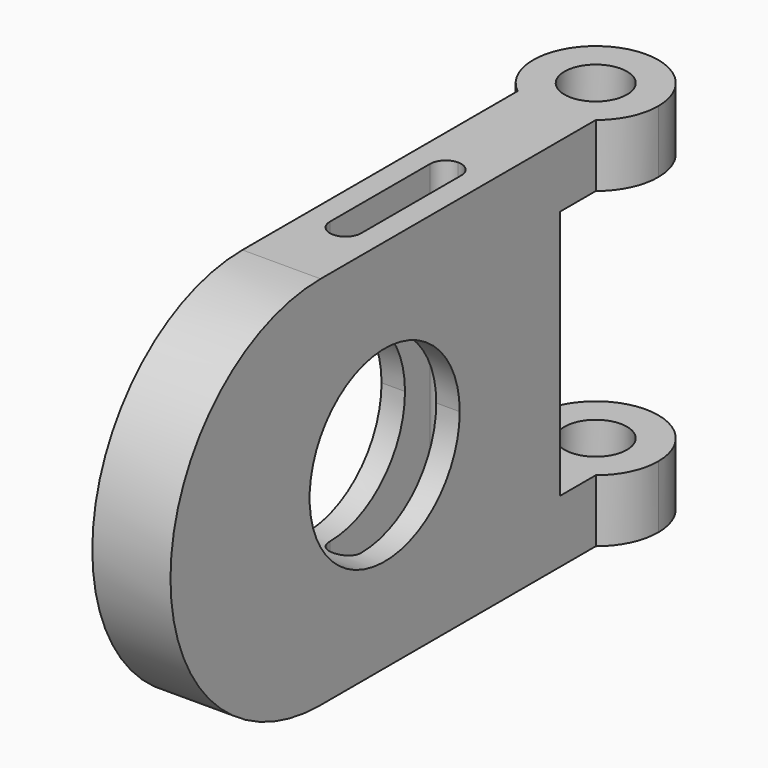
from build123d import *
from build123d import SkipClean  # not in build123d's __all__

# Parameters (mm, degrees)
F1_DEPTH = 152.4
F2_DEPTH = 25.4
F4_DEPTH = 31.75
F5_DEPTH = 41.276
F3_W     = 18.2721313551
F3_H     = 101.6
F6_DEPTH = 41.276
F8_DEPTH = 25.4


with BuildPart() as f1:
    # F0 (on Top) → F1 (new body)
    with BuildSketch(Plane.XY):
        with BuildLine():
            ThreePointArc((15.875, -7.1278686449), (8.4122570223, -11.266516889), (0, -12.7))
            ThreePointArc((0, -12.7), (-8.4122570223, -11.266516889), (-15.875, -7.1278686449))
            Line((-15.875, -7.1278686449), (-15.875, -146.8278686449))
            Line((-15.875, -146.8278686449), (15.875, -146.8278686449))
            Line((15.875, -146.8278686449), (15.875, -7.1278686449))
        make_face()
        with BuildLine():
            ThreePointArc((-6.35, -63.5), (-4.4901280605, -59.0098719395), (0, -57.15))
            ThreePointArc((0, -57.15), (4.4901280605, -59.0098719395), (6.35, -63.5))
            Line((6.35, -63.5), (6.35, -114.3))
            ThreePointArc((6.35, -114.3), (0, -120.65), (-6.35, -114.3))
            Line((-6.35, -114.3), (-6.35, -63.5))
        make_face(mode=Mode.SUBTRACT)
        with BuildLine():
            Line((15.875, -7.1278686449), (0, -7.1278686449))
            Line((0, -7.1278686449), (0, -12.7))
            ThreePointArc((0, -12.7), (8.4122570223, -11.266516889), (15.875, -7.1278686449))
        make_face()
        with BuildLine():
            Line((0, -12.7), (0, -7.1278686449))
            Line((0, -7.1278686449), (-15.875, -7.1278686449))
            ThreePointArc((-15.875, -7.1278686449), (-8.4122570223, -11.266516889), (0, -12.7))
        make_face()
    extrude(amount=-F1_DEPTH)

    # F0 (on Top) → F2 (join)
    with BuildSketch(Plane.XY):
        with BuildLine():
            Line((-15.875, -7.1278686449), (0, -7.1278686449))
            Line((0, -7.1278686449), (15.875, -7.1278686449))
            ThreePointArc((15.875, -7.1278686449), (22.8952505992, 1.7014773719), (25.4, 12.7))
            ThreePointArc((25.4, 12.7), (-10.9985226281, 35.5952505992), (-15.875, -7.1278686449))
        make_face()
        with BuildLine():
            ThreePointArc((12.7, 12.7), (8.9802561211, 3.7197438789), (0, 0))
            ThreePointArc((0, 0), (-8.9802561211, 21.6802561211), (12.7, 12.7))
        make_face(mode=Mode.SUBTRACT)
    extrude(amount=-F2_DEPTH)

    # F3 (on face) → F4 (join)
    with BuildSketch(Plane.YZ.offset(15.875)):
        with BuildLine():
            Line((-146.8278686449, -56.3619617548), (-146.8278686449, 0))
            ThreePointArc((-146.8278686449, 0), (-223.0278686449, -76.2), (-146.8278686449, -152.4))
            Line((-146.8278686449, -152.4), (-146.8278686449, -96.0380382452))
            ThreePointArc((-146.8278686449, -96.0380382452), (-152.4, -76.2), (-146.8278686449, -56.3619617548))
        make_face()
    extrude(amount=-F4_DEPTH)

    # F3 (on face) → F5 (cut, through all)
    with BuildSketch(Plane.YZ.offset(15.875)):
        with BuildLine():
            ThreePointArc((-76.2, -76.2), (-103.9971313551, -39.5194752261), (-146.8278686449, -56.3619617548))
            Line((-146.8278686449, -56.3619617548), (-146.8278686449, -96.0380382452))
            ThreePointArc((-146.8278686449, -96.0380382452), (-103.9971313551, -112.8805247739), (-76.2, -76.2))
        make_face()
    with SkipClean():  # cleaning this boolean's faces spoils the solid; the shape is the same uncleaned
        extrude(amount=-F5_DEPTH, mode=Mode.SUBTRACT)

    # F3 (on face) → F6 (cut, through all)
    with BuildSketch(Plane.YZ.offset(15.875)):
        with Locations((-16.2639343225, -76.2)):
            Rectangle(F3_W, F3_H)
    extrude(amount=-F6_DEPTH, mode=Mode.SUBTRACT)

    # F7 (on face) → F8 (join)
    with BuildSketch(Plane(origin=(0, 0, -152.4), x_dir=(1, 0, 0), z_dir=(0, 0, -1))):
        with BuildLine():
            ThreePointArc((-15.875, 7.1278686449), (-10.9985226281, -35.5952505992), (25.4, -12.7))
            ThreePointArc((25.4, -12.7), (22.8952505992, -1.7014773719), (15.875, 7.1278686449))
            Line((15.875, 7.1278686449), (-15.875, 7.1278686449))
        make_face()
        with BuildLine():
            ThreePointArc((0, 0), (8.9802561211, -3.7197438789), (12.7, -12.7))
            ThreePointArc((12.7, -12.7), (-8.9802561211, -21.6802561211), (0, 0))
        make_face(mode=Mode.SUBTRACT)
    extrude(amount=-F8_DEPTH)


solid = f1.part
